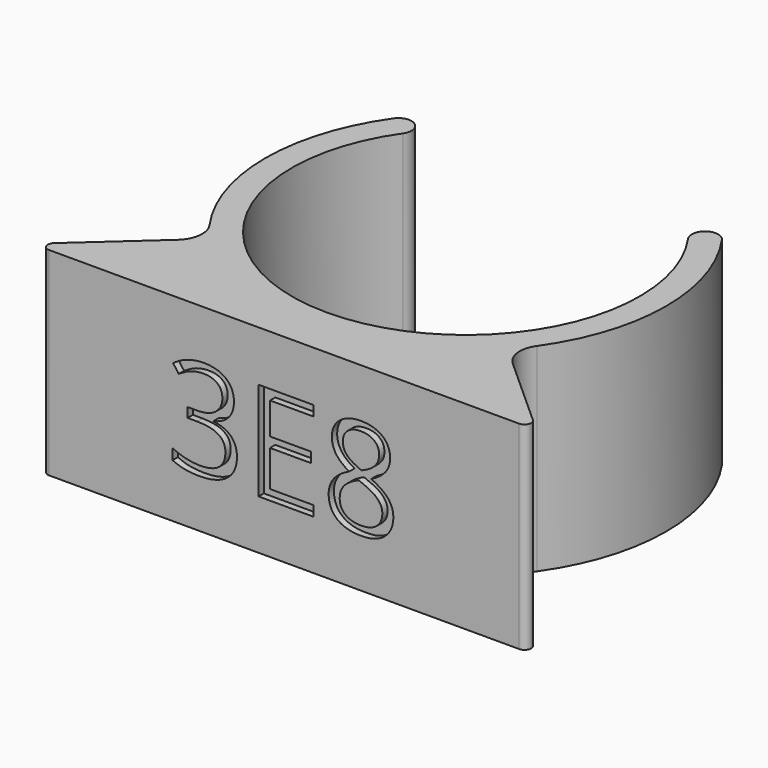
from build123d import *

# Parameters (mm, degrees)
F3_DEPTH     = 15
F4_R         = 2
F5_R         = 0.5
F6_TEXT_SIZE = 10.4166666667
F7_DEPTH     = 0.5


# Not quite as in the source:
# - Text() gives the source's letters only with a copy of the font that has no kerning and outlines rounded to 1/6400 em; it was checked with that copy


with BuildPart() as f3:
    # F2 (on Top) → F3 (new body)
    with BuildSketch(Plane.XY):
        with BuildLine():
            ThreePointArc((10.7718493824, 7.542530138), (0, -13.15), (-10.7718493824, 7.542530138))
            ThreePointArc((-10.7718493824, 7.542530138), (-11.0174249903, 8.9352586187), (-12.410153471, 8.6896830107))
            ThreePointArc((-12.410153471, 8.6896830107), (-15.1219789433, -0.9210064268), (-11.2638433283, -10.1315513854))
            ThreePointArc((-11.2638433283, -10.1315513854), (0, -15.15), (11.2638433283, -10.1315513854))
            ThreePointArc((11.2638433283, -10.1315513854), (15.1219789433, -0.9210064268), (12.410153471, 8.6896830107))
            ThreePointArc((12.410153471, 8.6896830107), (11.0174249903, 8.9352586187), (10.7718493824, 7.542530138))
        make_face()
        with BuildLine():
            ThreePointArc((11.2638433283, -10.1315513854), (0, -15.15), (-11.2638433283, -10.1315513854))
            Line((-11.2638433283, -10.1315513854), (-19.0666666667, -17.15))
            Line((-19.0666666667, -17.15), (19.0666666667, -17.15))
            Line((19.0666666667, -17.15), (11.2638433283, -10.1315513854))
        make_face()
    extrude(amount=F3_DEPTH)

    # F4
    f4_edges = [f3.edges().sort_by_distance(p)[0] for p in [
        (11.263843, -10.131551, 7.5),
        (-11.263843, -10.131551, 7.5),
    ]]
    fillet(f4_edges, radius=F4_R)

    # F5
    f5_edges = [f3.edges().sort_by_distance(p)[0] for p in [
        (-19.066667, -17.15, 7.5),
        (19.066667, -17.15, 7.5),
    ]]
    fillet(f5_edges, radius=F5_R)

    # F6 (on face) → F7 (cut)
    with BuildSketch(Plane.XZ.offset(17.15)):
        with Locations((-8.9200846354, 3.75)):
            Text('3E8', F6_TEXT_SIZE, font='Open Sans', text_align=(TextAlign.LEFT, TextAlign.BOTTOM))
    extrude(amount=-F7_DEPTH, mode=Mode.SUBTRACT)


solid = f3.part
